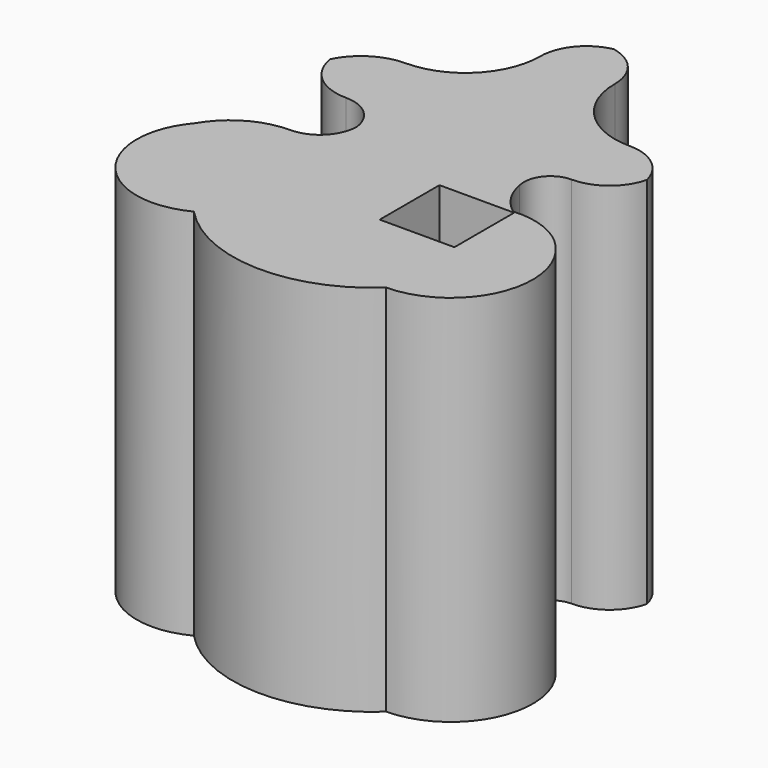
from build123d import *

# Parameters (mm, degrees)
F0_W     = 25.4
F0_H     = 25.4
F1_DEPTH = 63.5


with BuildPart() as f1:
    # F0 (on Top) → F1 (new body, symmetric)
    with BuildSketch(Plane.XY):
        with BuildLine():
            Line((-12.7, 58.4446051985), (0, 58.4446051985))
            Line((0, 58.4446051985), (12.7, 58.4446051985))
            ThreePointArc((12.7, 58.4446051985), (9.1177237853, 68.4465950708), (0, 73.8999992609))
            ThreePointArc((0, 73.8999992609), (-9.1177237853, 68.4465950708), (-12.7, 58.4446051985))
        make_face()
        Polygon((12.7, 58.4446051985), (0, 58.4446051985), (-12.7, 58.4446051985), (-12.7, 33.0446051985), (-38.1, 33.0446051985), (-38.1, 7.6446051985), (-12.7, 7.6446051985), (-12.7, -16.1055155754), (-12.7, -41.5055155754), (-12.7, -49.8682335019), (12.7, -49.8682335019), (12.7, -41.5055155754), (12.7, -16.1055155754), (12.7, 8.3362860605), (38.1, 8.3362860605), (38.1, 33.0446051985), (12.7, 33.0446051985), (12.7, 45.7446051985), align=None)
        with BuildLine():
            ThreePointArc((38.1, 33.0446051985), (20.1394877579, 40.4840929564), (12.7, 58.4446051985))
            Line((12.7, 58.4446051985), (12.7, 45.7446051985))
            Line((12.7, 45.7446051985), (12.7, 33.0446051985))
            Line((12.7, 33.0446051985), (38.1, 33.0446051985))
        make_face()
        with BuildLine():
            Line((-12.7, 33.0446051985), (-12.7, 58.4446051985))
            ThreePointArc((-12.7, 58.4446051985), (-20.1394877579, 40.4840929564), (-38.1, 33.0446051985))
            Line((-38.1, 33.0446051985), (-12.7, 33.0446051985))
        make_face()
        with BuildLine():
            ThreePointArc((53.8339801133, 20.6904456295), (48.1022920981, 29.5869981283), (38.1, 33.0446051985))
            Line((38.1, 33.0446051985), (38.1, 8.3362860605))
            ThreePointArc((38.1, 8.3362860605), (48.1022920981, 11.7938931307), (53.8339801133, 20.6904456295))
        make_face()
        with BuildLine():
            Line((-38.1, 7.6446051985), (-38.1, 33.0446051985))
            ThreePointArc((-38.1, 33.0446051985), (-48.1779241379, 30.1618280155), (-55.2068687975, 22.3856531084))
            ThreePointArc((-55.2068687975, 22.3856531084), (-49.3909637934, 11.8382480748), (-38.1, 7.6446051985))
        make_face()
        with BuildLine():
            ThreePointArc((29.4168628752, -3.037011018), (30.9454777105, 4.7972348951), (38.1, 8.3362860605))
            Line((38.1, 8.3362860605), (12.7, 8.3362860605))
            Line((12.7, 8.3362860605), (12.7, -16.1055155754))
            Line((12.7, -16.1055155754), (38.1, -16.1055155754))
            ThreePointArc((38.1, -16.1055155754), (37.8112363374, -15.9115868292), (37.5258770827, -15.7126825627))
            ThreePointArc((37.5258770827, -15.7126825627), (32.2384158105, -10.1636052268), (29.4168628752, -3.037011018))
        make_face()
        with BuildLine():
            Line((-12.7, 7.6446051985), (-38.1, 7.6446051985))
            ThreePointArc((-38.1, 7.6446051985), (-29.6939751713, 4.5068420563), (-25.4, -3.3715199679))
            ThreePointArc((-25.4, -3.3715199679), (-29.107716584, -12.3737471543), (-38.1, -16.1055155754))
            Line((-38.1, -16.1055155754), (-12.7, -16.1055155754))
            Line((-12.7, -16.1055155754), (-12.7, 7.6446051985))
        make_face()
        with BuildLine():
            ThreePointArc((60.5236142874, -26.4526233077), (50.436987874, -18.0585790132), (37.5258770827, -15.7126825627))
            ThreePointArc((37.5258770827, -15.7126825627), (37.8112363374, -15.9115868292), (38.1, -16.1055155754))
            Line((38.1, -16.1055155754), (38.1, -41.5055155754))
            Line((38.1, -41.5055155754), (12.7, -41.5055155754))
            Line((12.7, -41.5055155754), (12.7, -49.8682335019))
            Line((12.7, -49.8682335019), (-12.7, -49.8682335019))
            Line((-12.7, -49.8682335019), (-12.7, -41.5055155754))
            Line((-12.7, -41.5055155754), (-38.1, -41.5055155754))
            ThreePointArc((-38.1, -41.5055155754), (-37.9658127793, -56.6748011531), (-28.7389459174, -68.7159871021))
            ThreePointArc((-28.7389459174, -68.7159871021), (4.3955551034, -83.6780580167), (38.4478494525, -70.9422826767))
            ThreePointArc((38.4478494525, -70.9422826767), (63.1143336959, -55.4599639488), (60.5236142874, -26.4526233077))
        make_face()
        with Locations((-25.4, -28.8055155754)):
            Rectangle(F0_W, F0_H)
        with BuildLine():
            Line((-38.1, -41.5055155754), (-38.1, -16.1055155754))
            ThreePointArc((-38.1, -16.1055155754), (-50.8550498174, -19.5062062845), (-60.2240860462, -28.8055155754))
            ThreePointArc((-60.2240860462, -28.8055155754), (-50.8550498174, -38.1048248663), (-38.1, -41.5055155754))
        make_face()
        with BuildLine():
            ThreePointArc((-28.7389459174, -68.7159871021), (-37.9658127793, -56.6748011531), (-38.1, -41.5055155754))
            ThreePointArc((-38.1, -41.5055155754), (-50.8550498174, -38.1048248663), (-60.2240860462, -28.8055155754))
            ThreePointArc((-60.2240860462, -28.8055155754), (-60.9967813298, -61.7895486407), (-28.7389459174, -68.7159871021))
        make_face()
    extrude(amount=F1_DEPTH, both=True)


solid = f1.part
